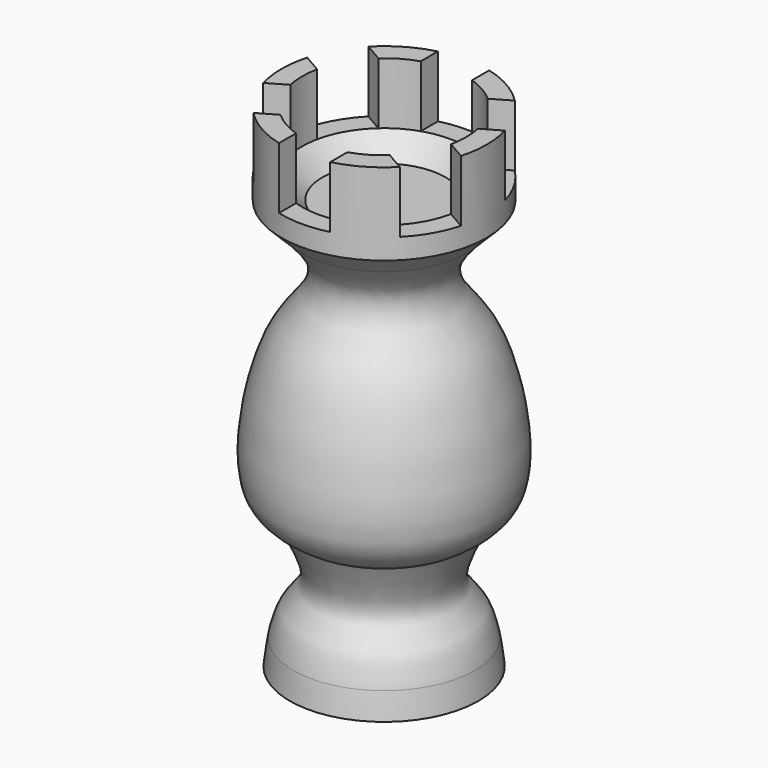
from build123d import *

# Parameters (mm, degrees)
F2_W            = 5
F2_H            = 30
F3_DEPTH        = 6
F3_COPIES_COUNT = 3
F3_COPIES_ANGLE = 120
F4_SIZE         = 1.99999


# Not quite as in the source:
# - a fillet or chamfer is up to 0.001 mm smaller than in the source, because OpenCascade refuses the exact size
# - a pattern or mirror of a feature is missing from the dataset's text; its kind, count and spacing are read off the source's solid


with BuildPart() as f1:
    # F0 (on Front) → F1 (revolve)
    with BuildSketch(Plane.XZ):
        Polygon((0, 40), (0, 38), (8, 38), (10, 40), (10, 48), (8, 48), (8, 40), align=None)
        with BuildLine():
            Line((0, 38), (0, 2.5))
            Line((0, 2.5), (8.8359999515, 2.5))
            add(Edge.make_bspline(
                [(8, 12.533579953), (7.0532389771, 10.6726538049), (5.3869298638, 7.3974046925), (8.0507795967, 5.5349261703), (8.6558075337, 3.4465494126), (8.8359999515, 2.5)],
                knots=[0, 0, 0, 0, 0.3637164633, 0.6401447069, 0.8357164003, 0.8357164003, 0.8357164003, 0.8357164003], degree=3))
            add(Edge.make_bspline(
                [(8, 38), (7.0589282052, 36.9435184781), (5.3143712589, 34.9850152183), (6.2355979215, 31.5927216769), (9.9148243241, 28.6346543207), (12.3503514137, 15.4330853755), (9.1906018857, 13.3271150713), (8, 12.533579953)],
                knots=[0, 0, 0, 0, 0.1718343327, 0.3185461304, 0.509446344, 0.8151580995, 1, 1, 1, 1], degree=3))
            Line((8, 38), (0, 38))
        make_face()
        with BuildLine():
            Line((0, 2.5), (0, 0))
            Line((0, 0), (9.1906018857, 0))
            add(Edge.make_bspline(
                [(8.8359999515, 2.5), (8.9873646942, 1.7048821478), (9.0889832899, 0.8524410739), (9.1906018857, 0)],
                knots=[0.8357164003, 0.8357164003, 0.8357164003, 0.8357164003, 1, 1, 1, 1], degree=3))
            Line((8.8359999515, 2.5), (0, 2.5))
        make_face()
    revolve(axis=Axis((0, 0, 24), (0, 0, 1)))

    # F2 (on face) → F3 (cut)
    with BuildSketch(Plane.XY.offset(48)):
        Rectangle(F2_W, F2_H)
    f3 = extrude(amount=-F3_DEPTH, mode=Mode.SUBTRACT)

    # F3_copies: F3 ×3 about axis
    f3_copies_axis = Axis((0, 0, 0), (0, 0, 1))
    for i in range(1, F3_COPIES_COUNT):
        add(f3.rotate(f3_copies_axis, i * F3_COPIES_ANGLE / (F3_COPIES_COUNT - 1)), mode=Mode.SUBTRACT)

    # F4 (size 2 in the source; OpenCascade refuses exactly that, so slightly less here)
    f4_edges = [f1.edges().sort_by_distance(p)[0] for p in [
        (-8, 0, 40),
    ]]
    chamfer(f4_edges, length=F4_SIZE)


solid = f1.part
